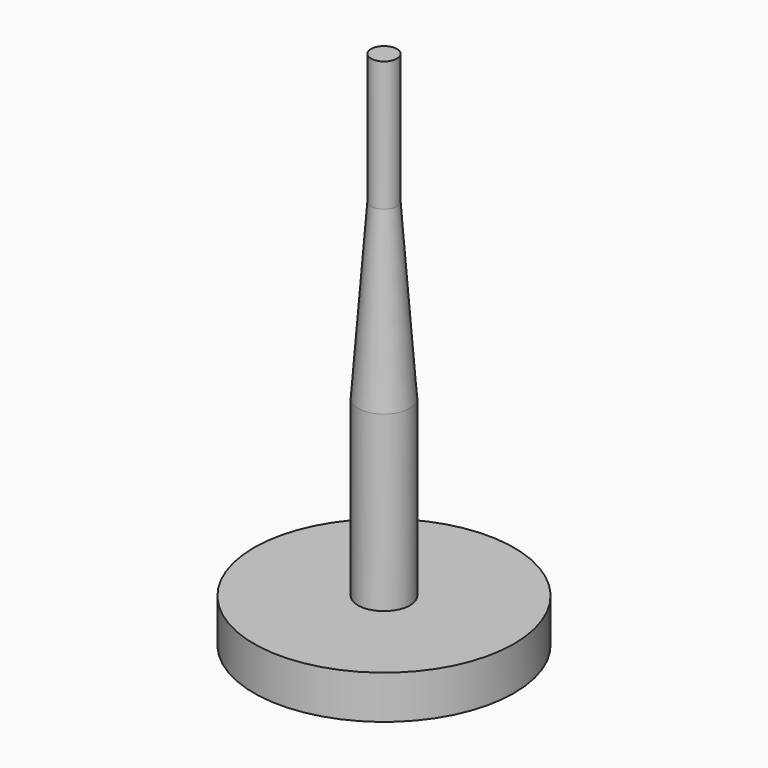
from build123d import *

# Parameters (mm, degrees)
F0_R     = 38.1
F1_DEPTH = 12.7
F2_R     = 7.62
F3_DEPTH = 50.8
F6_DEPTH = 38.1


# Not quite as in the source:
# - a feature names something its author has since deleted; it is built from what else it names


with BuildPart() as f1:
    # F0 (on Top) → F1 (new body)
    with BuildSketch(Plane.XY):
        Circle(F0_R)
    extrude(amount=F1_DEPTH)

    # F2 (on face) → F3 (join)
    with BuildSketch(Plane.XY.offset(12.7)):
        Circle(F2_R)
    extrude(amount=F3_DEPTH)

    # F4 (on Right) → F5 (revolve)
    with BuildSketch(Plane.YZ):
        Polygon((0, 114.3), (0, 63.5), (7.62, 63.5), (3.81, 114.3), align=None)
    revolve(axis=Axis((0, 0, 88.9), (0, 0, 1)))

    # F6 (add): a face of the model
    f6_faces = [f1.faces().sort_by_distance(p)[0] for p in [
        (0, 0, 114.3),
    ]]
    extrude(f6_faces, amount=F6_DEPTH)


solid = f1.part
